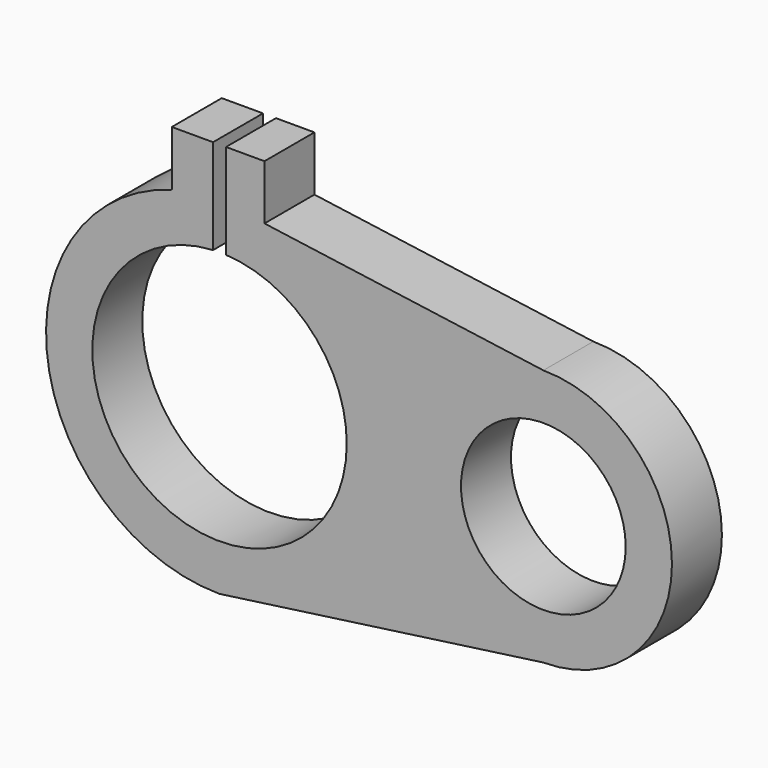
from build123d import *

# Parameters (mm, degrees)
F0_R     = 22.606
F1_DEPTH = 17.145


# Not quite as in the source:
# - a feature names something its author has since deleted; it is built from what else it names


with BuildPart() as f1:
    # F0 (on Front) → F1 (new body)
    with BuildSketch(Plane.XZ):
        with BuildLine():
            ThreePointArc((1.778, 34.8797124558), (25.3165190636, 24.0588754413), (34.925, 0))
            ThreePointArc((34.925, 0), (-24.0588754413, -25.3165190636), (-1.778, 34.8797124558))
            Line((-1.778, 34.8797124558), (-1.778, 47.591799094))
            ThreePointArc((-1.778, 47.591799094), (-7.4944029118, 47.0316335034), (-13.1017966196, 45.7873732631))
            ThreePointArc((-13.1017966196, 45.7873732631), (-47.1633558849, -6.6150197786), (0, -47.625))
            Line((0, -47.625), (88.9, -35.306))
            ThreePointArc((88.9, -35.306), (124.206, 0), (88.9, 35.306))
            Line((88.9, 35.306), (12.3385861516, 45.9152244904))
            Line((12.3385861516, 45.9152244904), (1.778, 47.37862))
            Line((1.778, 47.37862), (1.778, 34.8797124558))
        make_face()
        with Locations((88.9, 0)):
            Circle(F0_R, mode=Mode.SUBTRACT)
        with BuildLine():
            ThreePointArc((-13.1017966196, 45.7873732631), (-7.4944029118, 47.0316335034), (-1.778, 47.591799094))
            Line((-1.778, 47.591799094), (-1.778, 60.96))
            Line((-1.778, 60.96), (-13.1017966196, 60.96))
            Line((-13.1017966196, 60.96), (-13.1017966196, 45.7873732631))
        make_face()
        Polygon((1.778, 60.96), (1.778, 47.37862), (12.3385861516, 45.9152244904), (12.3385861516, 60.96), align=None)
    extrude(amount=F1_DEPTH)


solid = f1.part
